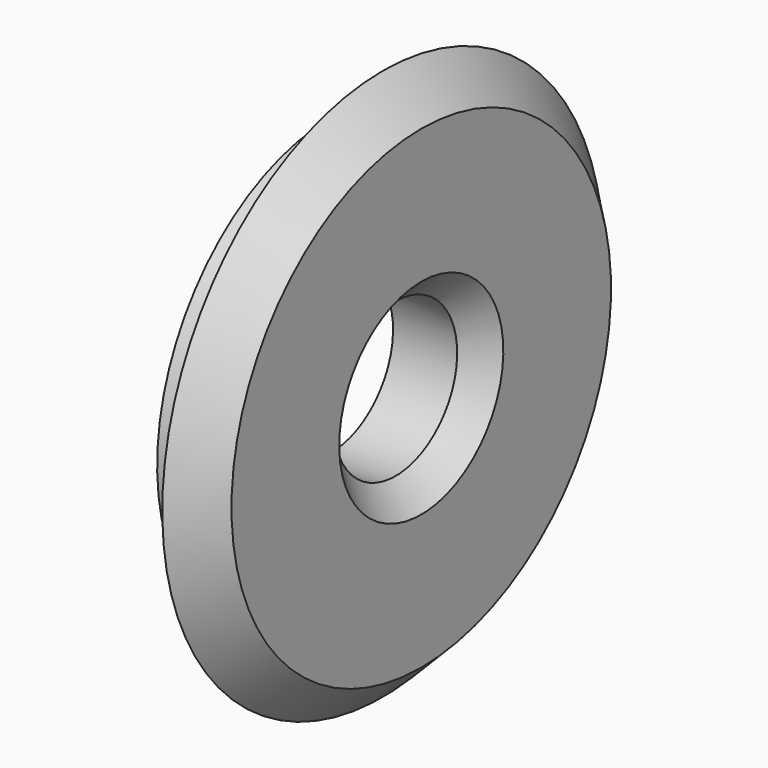
from build123d import *

# Parameters (mm, degrees)
F2_SIZE = 1
F3_SIZE = 1.49999


# Not quite as in the source:
# - a fillet or chamfer is up to 0.001 mm smaller than in the source, because OpenCascade refuses the exact size


with BuildPart() as f1:
    # F0 (on Front) → F1 (revolve)
    with BuildSketch(Plane.XZ):
        Polygon((0, 8.5), (0, 3), (3.5, 3), (3.5, 10.75), (2, 10.75), (2, 8.5), align=None)
    revolve(axis=Axis((1.1402515594, 0, 0), (1, 0, 0)))

    # F2
    f2_edges = [f1.edges().sort_by_distance(p)[0] for p in [
        (3.5, 0, -3),
    ]]
    chamfer(f2_edges, length=F2_SIZE)

    # F3 (size 1.5 in the source; OpenCascade refuses exactly that, so slightly less here)
    f3_edges = [f1.edges().sort_by_distance(p)[0] for p in [
        (3.5, 0, -10.75),
    ]]
    chamfer(f3_edges, length=F3_SIZE)


solid = f1.part
